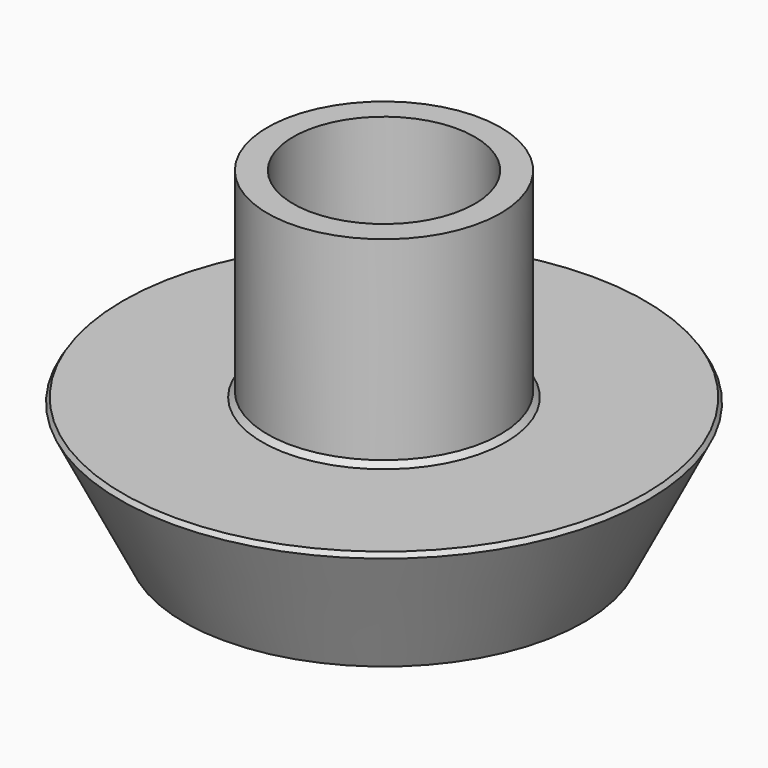
from build123d import *

# Parameters (mm, degrees)
F0_R          = 22.225
F0_R_2        = 17.315
F1_DEPTH      = 63.5
F4_SIZE       = 1
F5_R          = 4.9
F3_FACE_R     = 49.8
F3_FACE_R_2   = 22.225
F6_DEPTH      = 40
F7_DEPTH      = 63.501
F7_DEPTH_BACK = 30
F8_R          = 17.315
F9_DEPTH      = 12
F10_R         = 3
F11_R         = 33.5271440313
F12_DEPTH     = 7
F13_R         = 3
F14_W         = 5
F14_H         = 4.8698585015
F15_DEPTH     = 50.3537864045
F16_SIZE      = 1


# Not quite as in the source:
# - a feature names something its author has since deleted; it is built from what else it names


with BuildPart() as f1:
    # F0 (on Top) → F1 (new body)
    with BuildSketch(Plane.XY):
        Circle(F0_R)
        Circle(F0_R_2, mode=Mode.SUBTRACT)
    extrude(amount=F1_DEPTH)

    # F2 (on Right) → F3 (revolve)
    with BuildSketch(Plane.YZ):
        Polygon((-38.1, 0), (0, 0), (0, 25.4), (-17.315, 25.4), (-50.8, 25.4), align=None)
    revolve(axis=Axis((0, 0, 12.7), (0, 0, 1)))

    # F4
    f4_edges = [f1.edges().sort_by_distance(p)[0] for p in [
        (0, 50.8, 25.4),
    ]]
    chamfer(f4_edges, length=F4_SIZE)

    # F5 (on Top) + F3_face (on face) → F6 (cut)
    with BuildSketch(Plane.XY):
        Circle(F5_R)
    with BuildSketch(Plane.XY.offset(25.4)):
        Circle(F3_FACE_R)
        Circle(F3_FACE_R_2, mode=Mode.SUBTRACT)
    extrude(amount=F6_DEPTH, mode=Mode.SUBTRACT)

    # F5 (on Top) → F7 (cut, two sides)
    with BuildSketch(Plane.XY) as f7_sk:
        Circle(F5_R)
    extrude(amount=F7_DEPTH, mode=Mode.SUBTRACT)
    extrude(f7_sk.sketch, amount=-F7_DEPTH_BACK, mode=Mode.SUBTRACT)

    # F8 (on face) → F9 (cut)
    with BuildSketch(Plane.XY.offset(25.4)):
        Circle(F8_R)
    extrude(amount=-F9_DEPTH, mode=Mode.SUBTRACT)

    # F10
    f10_edges = [f1.edges().sort_by_distance(p)[0] for p in [
        (-17.315, 0, 13.4),
    ]]
    fillet(f10_edges, radius=F10_R)

    # F11 (on face) → F12 (cut)
    with BuildSketch(Plane(origin=(0, 0, 0), x_dir=(1, 0, 0), z_dir=(0, 0, -1))):
        Circle(F11_R)
    extrude(amount=-F12_DEPTH, mode=Mode.SUBTRACT)

    # F13
    f13_edges = [f1.edges().sort_by_distance(p)[0] for p in [
        (-33.527144, 0, 7),
    ]]
    fillet(f13_edges, radius=F13_R)

    # F14 (on Right) → F15 (cut, through all)
    with BuildSketch(Plane.YZ):
        with BuildLine():
            Line((-2.4888959483, 2.3854229395), (-2.5063311768, 0))
            Line((-2.5063311768, 0), (2.4936688232, 0))
            Line((2.4936688232, 0), (2.4921056953, 2.4222710093))
            ThreePointArc((2.4921056953, 2.4222710093), (0.0184938011, 0.120856929), (-2.4888959483, 2.3854229395))
        make_face()
        with Locations((-0.0063311768, -2.4349292507)):
            Rectangle(F14_W, F14_H)
        with BuildLine():
            Line((-2.485189612, 2.8925100588), (-2.4888959483, 2.3854229395))
            ThreePointArc((-2.4888959483, 2.3854229395), (0.0184938011, 0.120856929), (2.4921056953, 2.4222710093))
            Line((2.4921056953, 2.4222710093), (2.4918474071, 2.8225222584))
            ThreePointArc((2.4918474071, 2.8225222584), (0.0351518792, 5.1205413808), (-2.485189612, 2.8925100588))
        make_face()
        with BuildLine():
            ThreePointArc((-2.485189612, 2.8925100588), (-2.4999332245, 2.6390607164), (-2.4888959483, 2.3854229395))
            Line((-2.4888959483, 2.3854229395), (-2.485189612, 2.8925100588))
        make_face()
        with BuildLine():
            Line((2.4918474071, 2.8225222584), (2.4921056953, 2.4222710093))
            ThreePointArc((2.4921056953, 2.4222710093), (2.4980256442, 2.5214513158), (2.5, 2.6207885239))
            ThreePointArc((2.5, 2.6207885239), (2.4979610203, 2.7217377245), (2.4918474071, 2.8225222584))
        make_face()
    extrude(amount=-F15_DEPTH, mode=Mode.SUBTRACT)

    # F16
    f16_edges = [f1.edges().sort_by_distance(p)[0] for p in [
        (-22.225, 0, 25.4),
    ]]
    chamfer(f16_edges, length=F16_SIZE)


solid = f1.part
